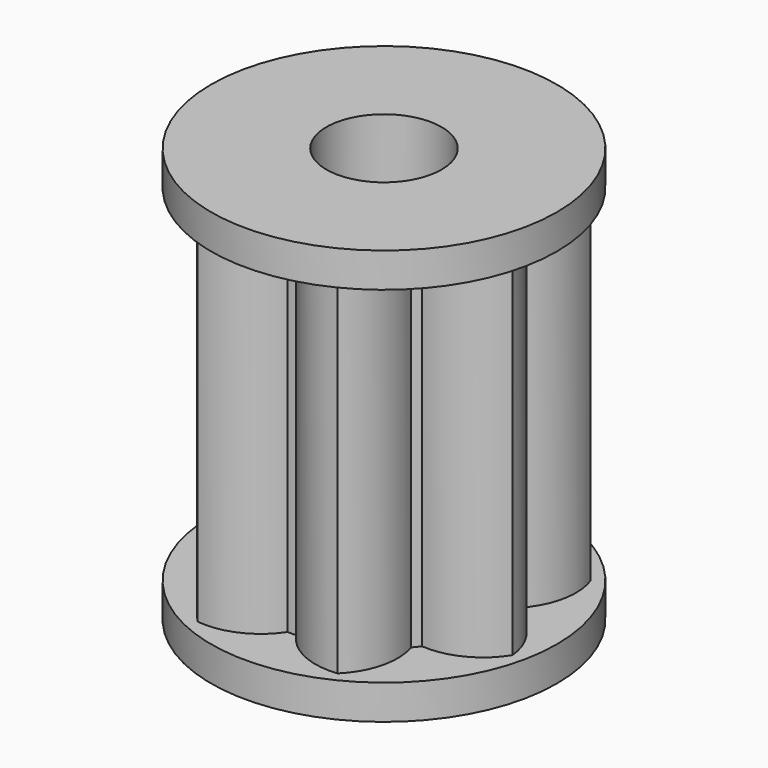
from build123d import *

# Parameters (mm, degrees)
F0_R     = 2.5
F1_DEPTH = 15
F2_R     = 7.5
F2_R_2   = 2.5
F3_DEPTH = 1.5
F4_R     = 7.5
F4_R_2   = 2.5
F5_DEPTH = 1.5


with BuildPart() as f1:
    # F0 (on Top) → F1 (new body)
    with BuildSketch(Plane.XY):
        with BuildLine():
            ThreePointArc((0, 7), (-1.3412127701, 6.0735823287), (-2, 4.582575695))
            ThreePointArc((-2, 4.582575695), (-2.1694186956, 4.5048443395), (-2.3358223454, 4.420852177))
            ThreePointArc((-2.3358223454, 4.420852177), (-3.9122853917, 4.8354190111), (-5.4728203773, 4.364428613))
            ThreePointArc((-5.4728203773, 4.364428613), (-5.5847503602, 2.7382142744), (-4.8297815528, 1.2935262471))
            ThreePointArc((-4.8297815528, 1.2935262471), (-4.8746395609, 1.1126046698), (-4.9127228226, 0.9301368008))
            ThreePointArc((-4.9127228226, 0.9301368008), (-6.2197528574, -0.0439134465), (-6.8244953853, -1.5576465377))
            ThreePointArc((-6.8244953853, -1.5576465377), (-5.622857021, -2.659084978), (-4.0226390868, -2.9695748479))
            ThreePointArc((-4.0226390868, -2.9695748479), (-3.9091574123, -3.1174490093), (-3.7902428131, -3.2609905577))
            ThreePointArc((-3.7902428131, -3.2609905577), (-3.8436195617, -4.8901781832), (-3.0371861738, -6.3067820753))
            ThreePointArc((-3.0371861738, -6.3067820753), (-1.4268376596, -6.0540390065), (-0.1863673415, -4.9965255142))
            ThreePointArc((-0.1863673415, -4.9965255142), (0, -5), (0.1863673415, -4.9965255142))
            ThreePointArc((0.1863673415, -4.9965255142), (1.4268376596, -6.0540390065), (3.0371861738, -6.3067820753))
            ThreePointArc((3.0371861738, -6.3067820753), (3.8436195617, -4.8901781832), (3.7902428131, -3.2609905577))
            ThreePointArc((3.7902428131, -3.2609905577), (3.9091574123, -3.1174490093), (4.0226390868, -2.9695748479))
            ThreePointArc((4.0226390868, -2.9695748479), (5.622857021, -2.659084978), (6.8244953853, -1.5576465377))
            ThreePointArc((6.8244953853, -1.5576465377), (6.2197528574, -0.0439134465), (4.9127228226, 0.9301368008))
            ThreePointArc((4.9127228226, 0.9301368008), (4.8746395609, 1.1126046698), (4.8297815528, 1.2935262471))
            ThreePointArc((4.8297815528, 1.2935262471), (5.5847503602, 2.7382142744), (5.4728203773, 4.364428613))
            ThreePointArc((5.4728203773, 4.364428613), (3.9122853917, 4.8354190111), (2.3358223454, 4.420852177))
            ThreePointArc((2.3358223454, 4.420852177), (2.1694186956, 4.5048443395), (2, 4.582575695))
            ThreePointArc((2, 4.582575695), (1.3412127701, 6.0735823287), (0, 7))
        make_face()
        Circle(F0_R, mode=Mode.SUBTRACT)
    extrude(amount=F1_DEPTH)

    # F2 (on face) → F3 (join)
    with BuildSketch(Plane.XY.offset(15)):
        Circle(F2_R)
        with BuildLine():
            ThreePointArc((4.8297815528, 1.2935262471), (4.8746395609, 1.1126046698), (4.9127228226, 0.9301368008))
            ThreePointArc((4.9127228226, 0.9301368008), (6.2197528574, -0.0439134465), (6.8244953853, -1.5576465377))
            ThreePointArc((6.8244953853, -1.5576465377), (5.622857021, -2.659084978), (4.0226390868, -2.9695748479))
            ThreePointArc((4.0226390868, -2.9695748479), (3.9091574123, -3.1174490093), (3.7902428131, -3.2609905577))
            ThreePointArc((3.7902428131, -3.2609905577), (3.8436195617, -4.8901781832), (3.0371861738, -6.3067820753))
            ThreePointArc((3.0371861738, -6.3067820753), (1.4268376596, -6.0540390065), (0.1863673415, -4.9965255142))
            ThreePointArc((0.1863673415, -4.9965255142), (0, -5), (-0.1863673415, -4.9965255142))
            ThreePointArc((-0.1863673415, -4.9965255142), (-1.4268376596, -6.0540390065), (-3.0371861738, -6.3067820753))
            ThreePointArc((-3.0371861738, -6.3067820753), (-3.8436195617, -4.8901781832), (-3.7902428131, -3.2609905577))
            ThreePointArc((-3.7902428131, -3.2609905577), (-3.9091574123, -3.1174490093), (-4.0226390868, -2.9695748479))
            ThreePointArc((-4.0226390868, -2.9695748479), (-5.622857021, -2.659084978), (-6.8244953853, -1.5576465377))
            ThreePointArc((-6.8244953853, -1.5576465377), (-6.2197528574, -0.0439134465), (-4.9127228226, 0.9301368008))
            ThreePointArc((-4.9127228226, 0.9301368008), (-4.8746395609, 1.1126046698), (-4.8297815528, 1.2935262471))
            ThreePointArc((-4.8297815528, 1.2935262471), (-5.5847503602, 2.7382142744), (-5.4728203773, 4.364428613))
            ThreePointArc((-5.4728203773, 4.364428613), (-3.9122853917, 4.8354190111), (-2.3358223454, 4.420852177))
            ThreePointArc((-2.3358223454, 4.420852177), (-2.1694186956, 4.5048443395), (-2, 4.582575695))
            ThreePointArc((-2, 4.582575695), (-1.3412127701, 6.0735823287), (0, 7))
            ThreePointArc((0, 7), (1.3412127701, 6.0735823287), (2, 4.582575695))
            ThreePointArc((2, 4.582575695), (2.1694186956, 4.5048443395), (2.3358223454, 4.420852177))
            ThreePointArc((2.3358223454, 4.420852177), (3.9122853917, 4.8354190111), (5.4728203773, 4.364428613))
            ThreePointArc((5.4728203773, 4.364428613), (5.5847503602, 2.7382142744), (4.8297815528, 1.2935262471))
        make_face(mode=Mode.SUBTRACT)
        with BuildLine():
            ThreePointArc((6.8244953853, -1.5576465377), (6.2197528574, -0.0439134465), (4.9127228226, 0.9301368008))
            ThreePointArc((4.9127228226, 0.9301368008), (4.8746395609, 1.1126046698), (4.8297815528, 1.2935262471))
            ThreePointArc((4.8297815528, 1.2935262471), (5.5847503602, 2.7382142744), (5.4728203773, 4.364428613))
            ThreePointArc((5.4728203773, 4.364428613), (3.9122853917, 4.8354190111), (2.3358223454, 4.420852177))
            ThreePointArc((2.3358223454, 4.420852177), (2.1694186956, 4.5048443395), (2, 4.582575695))
            ThreePointArc((2, 4.582575695), (1.3412127701, 6.0735823287), (0, 7))
            ThreePointArc((0, 7), (-1.3412127701, 6.0735823287), (-2, 4.582575695))
            ThreePointArc((-2, 4.582575695), (-2.1694186956, 4.5048443395), (-2.3358223454, 4.420852177))
            ThreePointArc((-2.3358223454, 4.420852177), (-3.9122853917, 4.8354190111), (-5.4728203773, 4.364428613))
            ThreePointArc((-5.4728203773, 4.364428613), (-5.5847503602, 2.7382142744), (-4.8297815528, 1.2935262471))
            ThreePointArc((-4.8297815528, 1.2935262471), (-4.8746395609, 1.1126046698), (-4.9127228226, 0.9301368008))
            ThreePointArc((-4.9127228226, 0.9301368008), (-6.2197528574, -0.0439134465), (-6.8244953853, -1.5576465377))
            ThreePointArc((-6.8244953853, -1.5576465377), (-5.622857021, -2.659084978), (-4.0226390868, -2.9695748479))
            ThreePointArc((-4.0226390868, -2.9695748479), (-3.9091574123, -3.1174490093), (-3.7902428131, -3.2609905577))
            ThreePointArc((-3.7902428131, -3.2609905577), (-3.8436195617, -4.8901781832), (-3.0371861738, -6.3067820753))
            ThreePointArc((-3.0371861738, -6.3067820753), (-1.4268376596, -6.0540390065), (-0.1863673415, -4.9965255142))
            ThreePointArc((-0.1863673415, -4.9965255142), (0, -5), (0.1863673415, -4.9965255142))
            ThreePointArc((0.1863673415, -4.9965255142), (1.4268376596, -6.0540390065), (3.0371861738, -6.3067820753))
            ThreePointArc((3.0371861738, -6.3067820753), (3.8436195617, -4.8901781832), (3.7902428131, -3.2609905577))
            ThreePointArc((3.7902428131, -3.2609905577), (3.9091574123, -3.1174490093), (4.0226390868, -2.9695748479))
            ThreePointArc((4.0226390868, -2.9695748479), (5.622857021, -2.659084978), (6.8244953853, -1.5576465377))
        make_face()
        Circle(F2_R_2, mode=Mode.SUBTRACT)
    extrude(amount=F3_DEPTH)

    # F4 (on face) → F5 (join)
    with BuildSketch(Plane(origin=(0, 0, 0), x_dir=(1, 0, 0), z_dir=(0, 0, -1))):
        Circle(F4_R)
        with BuildLine():
            ThreePointArc((4.9127228226, -0.9301368008), (4.8746395609, -1.1126046698), (4.8297815528, -1.2935262471))
            ThreePointArc((4.8297815528, -1.2935262471), (5.5847503602, -2.7382142744), (5.4728203773, -4.364428613))
            ThreePointArc((5.4728203773, -4.364428613), (3.9122853917, -4.8354190111), (2.3358223454, -4.420852177))
            ThreePointArc((2.3358223454, -4.420852177), (2.1694186956, -4.5048443395), (2, -4.582575695))
            ThreePointArc((2, -4.582575695), (1.3412127701, -6.0735823287), (0, -7))
            ThreePointArc((0, -7), (-1.3412127701, -6.0735823287), (-2, -4.582575695))
            ThreePointArc((-2, -4.582575695), (-2.1694186956, -4.5048443395), (-2.3358223454, -4.420852177))
            ThreePointArc((-2.3358223454, -4.420852177), (-3.9122853917, -4.8354190111), (-5.4728203773, -4.364428613))
            ThreePointArc((-5.4728203773, -4.364428613), (-5.5847503602, -2.7382142744), (-4.8297815528, -1.2935262471))
            ThreePointArc((-4.8297815528, -1.2935262471), (-4.8746395609, -1.1126046698), (-4.9127228226, -0.9301368008))
            ThreePointArc((-4.9127228226, -0.9301368008), (-6.2197528574, 0.0439134465), (-6.8244953853, 1.5576465377))
            ThreePointArc((-6.8244953853, 1.5576465377), (-5.622857021, 2.659084978), (-4.0226390868, 2.9695748479))
            ThreePointArc((-4.0226390868, 2.9695748479), (-3.9091574123, 3.1174490093), (-3.7902428131, 3.2609905577))
            ThreePointArc((-3.7902428131, 3.2609905577), (-3.8436195617, 4.8901781832), (-3.0371861738, 6.3067820753))
            ThreePointArc((-3.0371861738, 6.3067820753), (-1.4268376596, 6.0540390065), (-0.1863673415, 4.9965255142))
            ThreePointArc((-0.1863673415, 4.9965255142), (0, 5), (0.1863673415, 4.9965255142))
            ThreePointArc((0.1863673415, 4.9965255142), (1.4268376596, 6.0540390065), (3.0371861738, 6.3067820753))
            ThreePointArc((3.0371861738, 6.3067820753), (3.8436195617, 4.8901781832), (3.7902428131, 3.2609905577))
            ThreePointArc((3.7902428131, 3.2609905577), (3.9091574123, 3.1174490093), (4.0226390868, 2.9695748479))
            ThreePointArc((4.0226390868, 2.9695748479), (5.622857021, 2.659084978), (6.8244953853, 1.5576465377))
            ThreePointArc((6.8244953853, 1.5576465377), (6.2197528574, 0.0439134465), (4.9127228226, -0.9301368008))
        make_face(mode=Mode.SUBTRACT)
        with BuildLine():
            ThreePointArc((5.4728203773, -4.364428613), (5.5847503602, -2.7382142744), (4.8297815528, -1.2935262471))
            ThreePointArc((4.8297815528, -1.2935262471), (4.8746395609, -1.1126046698), (4.9127228226, -0.9301368008))
            ThreePointArc((4.9127228226, -0.9301368008), (6.2197528574, 0.0439134465), (6.8244953853, 1.5576465377))
            ThreePointArc((6.8244953853, 1.5576465377), (5.622857021, 2.659084978), (4.0226390868, 2.9695748479))
            ThreePointArc((4.0226390868, 2.9695748479), (3.9091574123, 3.1174490093), (3.7902428131, 3.2609905577))
            ThreePointArc((3.7902428131, 3.2609905577), (3.8436195617, 4.8901781832), (3.0371861738, 6.3067820753))
            ThreePointArc((3.0371861738, 6.3067820753), (1.4268376596, 6.0540390065), (0.1863673415, 4.9965255142))
            ThreePointArc((0.1863673415, 4.9965255142), (0, 5), (-0.1863673415, 4.9965255142))
            ThreePointArc((-0.1863673415, 4.9965255142), (-1.4268376596, 6.0540390065), (-3.0371861738, 6.3067820753))
            ThreePointArc((-3.0371861738, 6.3067820753), (-3.8436195617, 4.8901781832), (-3.7902428131, 3.2609905577))
            ThreePointArc((-3.7902428131, 3.2609905577), (-3.9091574123, 3.1174490093), (-4.0226390868, 2.9695748479))
            ThreePointArc((-4.0226390868, 2.9695748479), (-5.622857021, 2.659084978), (-6.8244953853, 1.5576465377))
            ThreePointArc((-6.8244953853, 1.5576465377), (-6.2197528574, 0.0439134465), (-4.9127228226, -0.9301368008))
            ThreePointArc((-4.9127228226, -0.9301368008), (-4.8746395609, -1.1126046698), (-4.8297815528, -1.2935262471))
            ThreePointArc((-4.8297815528, -1.2935262471), (-5.5847503602, -2.7382142744), (-5.4728203773, -4.364428613))
            ThreePointArc((-5.4728203773, -4.364428613), (-3.9122853917, -4.8354190111), (-2.3358223454, -4.420852177))
            ThreePointArc((-2.3358223454, -4.420852177), (-2.1694186956, -4.5048443395), (-2, -4.582575695))
            ThreePointArc((-2, -4.582575695), (-1.3412127701, -6.0735823287), (0, -7))
            ThreePointArc((0, -7), (1.3412127701, -6.0735823287), (2, -4.582575695))
            ThreePointArc((2, -4.582575695), (2.1694186956, -4.5048443395), (2.3358223454, -4.420852177))
            ThreePointArc((2.3358223454, -4.420852177), (3.9122853917, -4.8354190111), (5.4728203773, -4.364428613))
        make_face()
        Circle(F4_R_2, mode=Mode.SUBTRACT)
    extrude(amount=F5_DEPTH)


solid = f1.part
